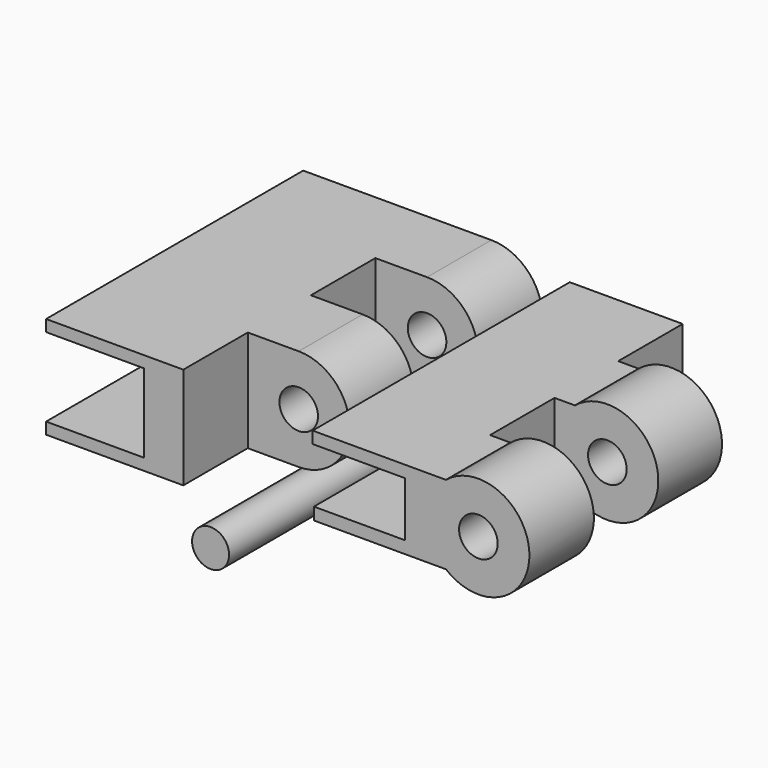
from build123d import *

# Parameters (mm, degrees)
F1_DEPTH  = 208.2
F3_D      = 25
F7_DEPTH  = 208.2
F9_D      = 25
F10_W     = 33.5077310764
F10_H     = 52.2
F10_W_2   = 41.4922689236
F10_W_3   = 42.0042114099
F10_W_4   = 32.9957885901
F10_W_5   = 75
F11_DEPTH = 66.0320122191
F12_W     = 75
F12_H     = 52.2
F13_DEPTH = 75
F14_R     = 12
F15_DEPTH = 230
F16_R     = 16.6914911111
F17_DEPTH = 15


with BuildPart() as f1:
    # F0 (on Front) → F1 (new body)
    with BuildSketch(Plane.XZ):
        with BuildLine():
            Line((5.9386579103, 34.0044003353), (-115.9613420897, 34.0044003353))
            Line((-115.9613420897, 34.0044003353), (-115.9613420897, 26.5044003353))
            Line((-115.9613420897, 26.5044003353), (-52.4613420897, 26.5044003353))
            Line((-52.4613420897, 26.5044003353), (-52.4613420897, -24.4955996647))
            Line((-52.4613420897, -24.4955996647), (-115.9613420897, -24.4955996647))
            Line((-115.9613420897, -24.4955996647), (-115.9613420897, -31.9955996647))
            Line((-115.9613420897, -31.9955996647), (5.9386579103, -31.9955996647))
            ThreePointArc((5.9386579103, -31.9955996647), (38.9386579103, 1.0044003353), (5.9386579103, 34.0044003353))
        make_face()
    extrude(amount=F1_DEPTH)

    # F3 (through all)
    with Locations(Plane(origin=(0, 0, 0), x_dir=(1, 0, 0), z_dir=(0, 1, 0))):
        with Locations((5.9386579103, -1.0044003353)):
            Hole(F3_D / 2)


with BuildPart() as f4_1:
    # F4: copy of F1
    add(f1.part.moved(Location((158.2, 0, 0))))


with BuildPart() as f7:
    # F5 (on face) → F7 (new body)
    with BuildSketch(Plane.XZ.offset(208.2)):
        with BuildLine():
            Line((143.0810586394, 26.5044003353), (56.7319393158, 26.5044003353))
            Line((56.7319393158, 26.5044003353), (56.7319393158, 18.8286447808))
            Line((56.7319393158, 18.8286447808), (116.6046112776, 18.8286447808))
            Line((116.6046112776, 18.8286447808), (116.6046112776, -16.5713552192))
            Line((116.6046112776, -16.5713552192), (57.5585439801, -16.5713552192))
            Line((57.5585439801, -16.5713552192), (57.5585439801, -24.4955996647))
            Line((57.5585439801, -24.4955996647), (143.0810586394, -24.4955996647))
            Line((143.0810586394, -24.4955996647), (143.0810586394, -24.4697121158))
            ThreePointArc((143.0810586394, -24.4697121158), (197.1386579103, 1.0044003353), (143.0810586394, 26.4785127863))
            Line((143.0810586394, 26.4785127863), (143.0810586394, 26.5044003353))
        make_face()
    extrude(amount=-F7_DEPTH)

    # F9 (through all)
    with Locations(Plane.XZ.offset(208.2)):
        with Locations((164.1076456912, 1.0044003353)):
            Hole(F9_D / 2)

    # F12 (on face) → F13 (cut, symmetric)
    with BuildSketch(Plane(origin=(0, 0, -24.4955996647), x_dir=(1, 0, 0), z_dir=(0, 0, -1))):
        with Locations((167.3975795507, 26.1)):
            Rectangle(F12_W, F12_H)
        with Locations((167.3975776881, 129.8699952722)):
            Rectangle(F12_W, F12_H)
    extrude(amount=F13_DEPTH, both=True, mode=Mode.SUBTRACT)


with BuildPart() as f1_1:
    add(f1.part)

    # F10 (on face) → F11 (cut, through all)
    with BuildSketch(Plane.XY.offset(34.0044003353)):
        with Locations((-10.8152076279, -78.15)):
            Rectangle(F10_W, F10_H)
        with Locations((26.6847923721, -78.15)):
            Rectangle(F10_W_2, F10_H)
        with Locations((26.9407636153, -182.1)):
            Rectangle(F10_W_3, F10_H)
        with Locations((-10.5592363847, -182.1)):
            Rectangle(F10_W_4, F10_H)
        with Locations((167.2925822881, -182.1)):
            Rectangle(F10_W_5, F10_H)
    extrude(amount=-F11_DEPTH, mode=Mode.SUBTRACT)


with BuildPart() as f15:
    # F14 (on Front) → F15 (new body)
    with BuildSketch(Plane.XZ):
        with Locations((8.0419126898, -47.4503040314)):
            Circle(F14_R)
    extrude(amount=F15_DEPTH)


with BuildPart() as f17:
    # F16 (on Front) → F17 (new body)
    with BuildSketch(Plane.XZ):
        with Locations((7.9846158624, -47.6694740355)):
            Circle(F16_R)
    extrude(amount=-F17_DEPTH)


solid = Compound([f7.part, f1_1.part, f15.part, f17.part])
